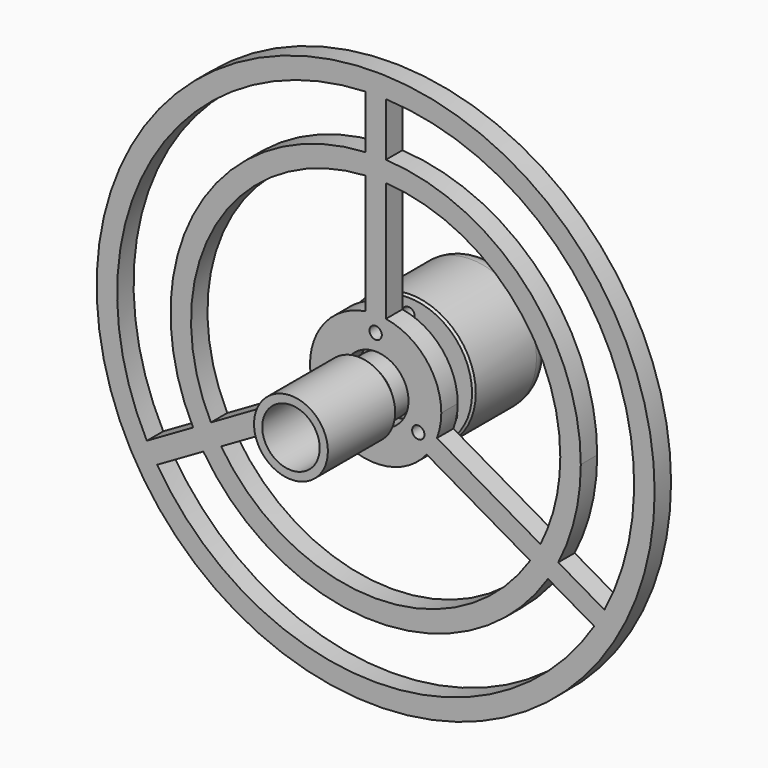
from build123d import *

# Parameters (mm, degrees)
F0_R           = 16
F0_R_2         = 1.5
F0_R_3         = 8
F1_DEPTH       = 24
F2_DEPTH       = 4
F3_DEPTH       = 2.8
F5_DEPTH       = 7.5
F6_R           = 5
F7_SIZE        = 0.5
F9_START       = 5
F8_R           = 7
F9_DEPTH       = 10
F10_R          = 9
F10_R_2        = 7
F11_DEPTH      = 18
F11_DEPTH_BACK = 5
F12_S5_R       = 7
F12_T6_DEPTH   = 14
F14_R          = 68
F14_R_2        = 1.5
F15_DEPTH      = 5


# Not quite as in the source:
# - a fillet or chamfer that OpenCascade refuses, or shapes differently, is made with other operations: its cross-section is extruded or revolved along the edge and cut away or added


with BuildPart() as f1:
    # F0 (on Front) → F1 (new body)
    with BuildSketch(Plane.XZ):
        Circle(F0_R)
        with Locations((-10.3923048454, -6)):
            Circle(F0_R_2, mode=Mode.SUBTRACT)
        with Locations((10.3923048454, -6)):
            Circle(F0_R_2, mode=Mode.SUBTRACT)
        Circle(F0_R_3, mode=Mode.SUBTRACT)
        with Locations((0, 12)):
            Circle(F0_R_2, mode=Mode.SUBTRACT)
        Circle(F0_R_3)
        with BuildLine():
            ThreePointArc((1.1989578808, 2.75), (2.5096686676, 1.6436432638), (3, 0))
            ThreePointArc((3, 0), (-1.6436432638, -2.5096686676), (-1.1989578808, 2.75))
            ThreePointArc((-1.1989578808, 2.75), (0, 3), (1.1989578808, 2.75))
        make_face(mode=Mode.SUBTRACT)
        with Locations((10.3923048454, -6)):
            Circle(F0_R_2)
        with Locations((-10.3923048454, -6)):
            Circle(F0_R_2)
        with Locations((0, 12)):
            Circle(F0_R_2)
        with BuildLine():
            Line((-1.1989578808, 2.75), (1.1989578808, 2.75))
            ThreePointArc((1.1989578808, 2.75), (0, 3), (-1.1989578808, 2.75))
        make_face()
        with BuildLine():
            ThreePointArc((-1.1989578808, 2.75), (-1.6436432638, -2.5096686676), (3, 0))
            ThreePointArc((3, 0), (2.5096686676, 1.6436432638), (1.1989578808, 2.75))
            Line((1.1989578808, 2.75), (-1.1989578808, 2.75))
        make_face()
    extrude(amount=-F1_DEPTH)

    # F0 (on Front) → F2 (cut)
    with BuildSketch(Plane.XZ):
        with Locations((-10.3923048454, -6)):
            Circle(F0_R_2)
        with Locations((0, 12)):
            Circle(F0_R_2)
        with Locations((10.3923048454, -6)):
            Circle(F0_R_2)
    extrude(amount=-F2_DEPTH, mode=Mode.SUBTRACT)

    # F0 (on Front) → F3 (join)
    with BuildSketch(Plane.XZ):
        with BuildLine():
            Line((-1.1989578808, 2.75), (1.1989578808, 2.75))
            ThreePointArc((1.1989578808, 2.75), (0, 3), (-1.1989578808, 2.75))
        make_face()
        with BuildLine():
            ThreePointArc((-1.1989578808, 2.75), (-1.6436432638, -2.5096686676), (3, 0))
            ThreePointArc((3, 0), (2.5096686676, 1.6436432638), (1.1989578808, 2.75))
            Line((1.1989578808, 2.75), (-1.1989578808, 2.75))
        make_face()
    extrude(amount=F3_DEPTH)

    # F4 (on face) → F5 (join)
    with BuildSketch(Plane.XZ.offset(2.8)):
        with BuildLine():
            ThreePointArc((-1.1989578808, 2.75), (-1.6436432638, -2.5096686676), (3, 0))
            ThreePointArc((3, 0), (2.5096686676, 1.6436432638), (1.1989578808, 2.75))
            Line((1.1989578808, 2.75), (-1.1989578808, 2.75))
        make_face()
    extrude(amount=F5_DEPTH)

    # F6
    f6_edges = [f1.edges().sort_by_distance(p)[0] for p in [
        (-16, 24, 0),
    ]]
    fillet(f6_edges, radius=F6_R)

    # F7
    f7_edges = [f1.edges().sort_by_distance(p)[0] for p in [
        (-16, 0, 0),
    ]]
    chamfer(f7_edges, length=F7_SIZE)


with BuildPart() as f9:
    # F8 (on face) → F9 (new body)
    with BuildSketch(Plane.XZ.offset(2.8).offset(F9_START)):
        Circle(F8_R)
        with BuildLine():
            ThreePointArc((1.1989578808, 2.75), (2.5096686676, 1.6436432638), (3, 0))
            ThreePointArc((3, 0), (-1.6436432638, -2.5096686676), (-1.1989578808, 2.75))
            ThreePointArc((-1.1989578808, 2.75), (0, 3), (1.1989578808, 2.75))
        make_face(mode=Mode.SUBTRACT)
        with BuildLine():
            Line((-1.1989578808, 2.75), (1.1989578808, 2.75))
            ThreePointArc((1.1989578808, 2.75), (0, 3), (-1.1989578808, 2.75))
        make_face()
    extrude(amount=F9_DEPTH)

    # F10 (on face) → F11 (join, two sides)
    with BuildSketch(Plane.XZ.offset(17.8)) as f11_sk:
        Circle(F10_R)
        Circle(F10_R_2, mode=Mode.SUBTRACT)
    extrude(amount=F11_DEPTH)
    extrude(f11_sk.sketch, amount=-F11_DEPTH_BACK)

    # F12: chamfer of 2.5 on 1 edges, made by hand


with BuildPart() as f12_tool2:
    # F12_s3 → F12_t4 (revolve)
    with BuildSketch(Plane.XY):
        Polygon((6.5, -12.8), (9, -15.3), (9, -12.8), align=None)
    revolve(axis=Axis((0, -12.8, 0), (0, -1, 0)))

    # F12_s5 → F12_t6 (cut, symmetric)
    with BuildSketch(Plane.XZ.offset(14)):
        Circle(F12_S5_R)
    extrude(amount=F12_T6_DEPTH, both=True, mode=Mode.SUBTRACT)


with BuildPart() as f9_1:
    add(f9.part)

    # F12_t1: cut F12_tool2
    add(f12_tool2.part, mode=Mode.SUBTRACT)


with BuildPart() as f15:
    # F14 (on offset) → F15 (new body)
    with BuildSketch(Plane.XZ.offset(5)):
        Circle(F14_R)
        with BuildLine():
            Line((2.5, 65.9391838022), (2.5, 62.9503772824))
            ThreePointArc((2.5, 62.9503772824), (45.4230117892, 43.6548966326), (63, 0))
            ThreePointArc((63, 0), (61.1649304421, -15.0947435888), (55.7666259044, -29.3101251318))
            Line((55.7666259044, -29.3101251318), (58.3550082775, -30.8045283916))
            Line((58.3550082775, -30.8045283916), (55.8550082775, -35.1346554106))
            Line((55.8550082775, -35.1346554106), (53.2666259044, -33.6402521507))
            ThreePointArc((53.2666259044, -33.6402521507), (0, -63), (-53.2666259044, -33.6402521507))
            Line((-53.2666259044, -33.6402521507), (-55.8550082775, -35.1346554106))
            Line((-55.8550082775, -35.1346554106), (-58.3550082775, -30.8045283916))
            Line((-58.3550082775, -30.8045283916), (-55.7666259044, -29.3101251318))
            ThreePointArc((-55.7666259044, -29.3101251318), (-54.5596004384, 31.5), (-2.5, 62.9503772824))
            Line((-2.5, 62.9503772824), (-2.5, 65.9391838022))
            Line((-2.5, 65.9391838022), (2.5, 65.9391838022))
        make_face(mode=Mode.SUBTRACT)
        with BuildLine():
            ThreePointArc((-40.1609560407, -20.3001874351), (-38.9711431703, 22.5), (-2.5, 44.930501889))
            Line((-2.5, 44.930501889), (-2.5, 49.9374608886))
            ThreePointArc((-2.5, 49.9374608886), (-43.3012701892, 25), (-44.49710973, -22.8036669348))
            Line((-44.49710973, -22.8036669348), (-40.1609560407, -20.3001874351))
        make_face()
        with BuildLine():
            Line((41.99710973, -27.1337939538), (37.6609560407, -24.630314454))
            ThreePointArc((37.6609560407, -24.630314454), (0, -45), (-37.6609560407, -24.630314454))
            Line((-37.6609560407, -24.630314454), (-41.99710973, -27.1337939538))
            ThreePointArc((-41.99710973, -27.1337939538), (0, -50), (41.99710973, -27.1337939538))
        make_face()
        with BuildLine():
            Line((2.5, 49.9374608886), (2.5, 44.930501889))
            ThreePointArc((2.5, 44.930501889), (32.6917420766, 30.9232921921), (45, 0))
            ThreePointArc((45, 0), (43.7735252283, -10.4344855688), (40.1609560407, -20.3001874351))
            Line((40.1609560407, -20.3001874351), (44.49710973, -22.8036669348))
            ThreePointArc((44.49710973, -22.8036669348), (48.6048119351, -11.729120033), (50, 0))
            ThreePointArc((50, 0), (36.2284418655, 34.4601218802), (2.5, 49.9374608886))
        make_face()
        with BuildLine():
            ThreePointArc((14.9362156932, -5.7366768052), (15.7318061756, -2.9172374697), (16, 0))
            ThreePointArc((16, 0), (12.1655250606, 10.3923048454), (2.5, 15.8034806293))
            Line((2.5, 15.8034806293), (2.5, 7.5993420768))
            ThreePointArc((2.5, 7.5993420768), (6.4807406984, 4.6904157598), (8, 0))
            ThreePointArc((8, 0), (7.9576939601, -0.8216488531), (7.8312232905, -1.6346075289))
            Line((7.8312232905, -1.6346075289), (14.9362156932, -5.7366768052))
        make_face()
        with BuildLine():
            Line((-2.5, 7.5993420768), (-2.5, 15.8034806293))
            ThreePointArc((-2.5, 15.8034806293), (-13.8564064606, 8), (-14.9362156932, -5.7366768052))
            Line((-14.9362156932, -5.7366768052), (-7.8312232905, -1.6346075289))
            ThreePointArc((-7.8312232905, -1.6346075289), (-6.9282032303, 4), (-2.5, 7.5993420768))
        make_face()
        with BuildLine():
            ThreePointArc((-12.4362156932, -10.0668038241), (0, -16), (12.4362156932, -10.0668038241))
            Line((12.4362156932, -10.0668038241), (5.3312232905, -5.9647345479))
            ThreePointArc((5.3312232905, -5.9647345479), (0, -8), (-5.3312232905, -5.9647345479))
            Line((-5.3312232905, -5.9647345479), (-12.4362156932, -10.0668038241))
        make_face()
        with BuildLine():
            ThreePointArc((-12.4362156932, -10.0668038241), (-13.8564064606, -8), (-14.9362156932, -5.7366768052))
            Line((-14.9362156932, -5.7366768052), (-40.1609560407, -20.3001874351))
            ThreePointArc((-40.1609560407, -20.3001874351), (-38.9711431703, -22.5), (-37.6609560407, -24.630314454))
            Line((-37.6609560407, -24.630314454), (-12.4362156932, -10.0668038241))
        make_face()
        with BuildLine():
            Line((40.1609560407, -20.3001874351), (14.9362156932, -5.7366768052))
            ThreePointArc((14.9362156932, -5.7366768052), (13.8564064606, -8), (12.4362156932, -10.0668038241))
            Line((12.4362156932, -10.0668038241), (37.6609560407, -24.630314454))
            ThreePointArc((37.6609560407, -24.630314454), (38.9711431703, -22.5), (40.1609560407, -20.3001874351))
        make_face()
        with BuildLine():
            ThreePointArc((-2.5, 15.8034806293), (0, 16), (2.5, 15.8034806293))
            Line((2.5, 15.8034806293), (2.5, 44.930501889))
            ThreePointArc((2.5, 44.930501889), (0, 45), (-2.5, 44.930501889))
            Line((-2.5, 44.930501889), (-2.5, 15.8034806293))
        make_face()
        with BuildLine():
            ThreePointArc((-41.99710973, -27.1337939538), (-43.3012701892, -25), (-44.49710973, -22.8036669348))
            Line((-44.49710973, -22.8036669348), (-55.7666259044, -29.3101251318))
            ThreePointArc((-55.7666259044, -29.3101251318), (-54.5596004384, -31.5), (-53.2666259044, -33.6402521507))
            Line((-53.2666259044, -33.6402521507), (-41.99710973, -27.1337939538))
        make_face()
        with BuildLine():
            Line((55.7666259044, -29.3101251318), (44.49710973, -22.8036669348))
            ThreePointArc((44.49710973, -22.8036669348), (43.3012701892, -25), (41.99710973, -27.1337939538))
            Line((41.99710973, -27.1337939538), (53.2666259044, -33.6402521507))
            ThreePointArc((53.2666259044, -33.6402521507), (54.5596004384, -31.5), (55.7666259044, -29.3101251318))
        make_face()
        with BuildLine():
            ThreePointArc((-2.5, 49.9374608886), (0, 50), (2.5, 49.9374608886))
            Line((2.5, 49.9374608886), (2.5, 62.9503772824))
            ThreePointArc((2.5, 62.9503772824), (0, 63), (-2.5, 62.9503772824))
            Line((-2.5, 62.9503772824), (-2.5, 49.9374608886))
        make_face()
        with BuildLine():
            Line((2.5, 7.5993420768), (2.5, 15.8034806293))
            ThreePointArc((2.5, 15.8034806293), (0, 16), (-2.5, 15.8034806293))
            Line((-2.5, 15.8034806293), (-2.5, 7.5993420768))
            ThreePointArc((-2.5, 7.5993420768), (0, 8), (2.5, 7.5993420768))
        make_face()
        with Locations((0, 12)):
            Circle(F14_R_2, mode=Mode.SUBTRACT)
        with BuildLine():
            Line((-7.8312232905, -1.6346075289), (-14.9362156932, -5.7366768052))
            ThreePointArc((-14.9362156932, -5.7366768052), (-13.8564064606, -8), (-12.4362156932, -10.0668038241))
            Line((-12.4362156932, -10.0668038241), (-5.3312232905, -5.9647345479))
            ThreePointArc((-5.3312232905, -5.9647345479), (-6.9282032303, -4), (-7.8312232905, -1.6346075289))
        make_face()
        with Locations((-10.3923048454, -6)):
            Circle(F14_R_2, mode=Mode.SUBTRACT)
        with BuildLine():
            ThreePointArc((12.4362156932, -10.0668038241), (13.8564064606, -8), (14.9362156932, -5.7366768052))
            Line((14.9362156932, -5.7366768052), (7.8312232905, -1.6346075289))
            ThreePointArc((7.8312232905, -1.6346075289), (6.9282032303, -4), (5.3312232905, -5.9647345479))
            Line((5.3312232905, -5.9647345479), (12.4362156932, -10.0668038241))
        make_face()
        with Locations((10.3923048454, -6)):
            Circle(F14_R_2, mode=Mode.SUBTRACT)
        with BuildLine():
            ThreePointArc((-37.6609560407, -24.630314454), (-38.9711431703, -22.5), (-40.1609560407, -20.3001874351))
            Line((-40.1609560407, -20.3001874351), (-44.49710973, -22.8036669348))
            ThreePointArc((-44.49710973, -22.8036669348), (-43.3012701892, -25), (-41.99710973, -27.1337939538))
            Line((-41.99710973, -27.1337939538), (-37.6609560407, -24.630314454))
        make_face()
        with BuildLine():
            Line((44.49710973, -22.8036669348), (40.1609560407, -20.3001874351))
            ThreePointArc((40.1609560407, -20.3001874351), (38.9711431703, -22.5), (37.6609560407, -24.630314454))
            Line((37.6609560407, -24.630314454), (41.99710973, -27.1337939538))
            ThreePointArc((41.99710973, -27.1337939538), (43.3012701892, -25), (44.49710973, -22.8036669348))
        make_face()
        with BuildLine():
            ThreePointArc((-2.5, 44.930501889), (0, 45), (2.5, 44.930501889))
            Line((2.5, 44.930501889), (2.5, 49.9374608886))
            ThreePointArc((2.5, 49.9374608886), (0, 50), (-2.5, 49.9374608886))
            Line((-2.5, 49.9374608886), (-2.5, 44.930501889))
        make_face()
        with BuildLine():
            ThreePointArc((-2.5, 62.9503772824), (0, 63), (2.5, 62.9503772824))
            Line((2.5, 62.9503772824), (2.5, 65.9391838022))
            Line((2.5, 65.9391838022), (-2.5, 65.9391838022))
            Line((-2.5, 65.9391838022), (-2.5, 62.9503772824))
        make_face()
        with BuildLine():
            ThreePointArc((-53.2666259044, -33.6402521507), (-54.5596004384, -31.5), (-55.7666259044, -29.3101251318))
            Line((-55.7666259044, -29.3101251318), (-58.3550082775, -30.8045283916))
            Line((-58.3550082775, -30.8045283916), (-55.8550082775, -35.1346554106))
            Line((-55.8550082775, -35.1346554106), (-53.2666259044, -33.6402521507))
        make_face()
        with BuildLine():
            Line((58.3550082775, -30.8045283916), (55.7666259044, -29.3101251318))
            ThreePointArc((55.7666259044, -29.3101251318), (54.5596004384, -31.5), (53.2666259044, -33.6402521507))
            Line((53.2666259044, -33.6402521507), (55.8550082775, -35.1346554106))
            Line((55.8550082775, -35.1346554106), (58.3550082775, -30.8045283916))
        make_face()
    extrude(amount=F15_DEPTH)


solid = Compound([f1.part, f9_1.part, f15.part])
